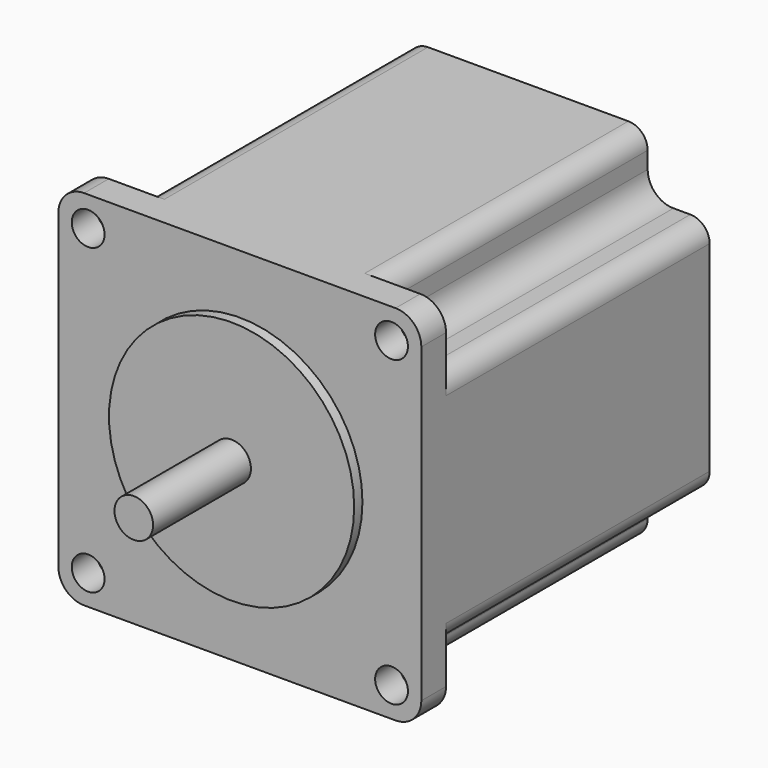
from build123d import *

# Parameters (mm, degrees)
F0_W     = 56.4
F0_H     = 56.4
F0_R     = 2.55
F0_R_2   = 19.05
F0_R_3   = 3
F1_DEPTH = 4.8
F2_DEPTH = 1.6
F3_DEPTH = 20.6
F4_R     = 4
F7_W     = 37.14
F7_H     = 9.63
F7_H_2   = 37.14
F7_W_2   = 9.63
F8_DEPTH = 56
F9_R     = 4
F10_R    = 3


# Not quite as in the source:
# - a feature of the source that left no trace in its solid (it failed there, or was rolled back) is left out


with BuildPart() as f1:
    # F0 (on Front) → F1 (new body)
    with BuildSketch(Plane.XZ):
        Rectangle(F0_W, F0_H)
        with Locations((-23.57, -23.57)):
            Circle(F0_R, mode=Mode.SUBTRACT)
        with Locations((23.57, -23.57)):
            Circle(F0_R, mode=Mode.SUBTRACT)
        with Locations((-23.57, 23.57)):
            Circle(F0_R, mode=Mode.SUBTRACT)
        Circle(F0_R_2, mode=Mode.SUBTRACT)
        with Locations((23.57, 23.57)):
            Circle(F0_R, mode=Mode.SUBTRACT)
        Circle(F0_R_2)
        Circle(F0_R_3, mode=Mode.SUBTRACT)
        Circle(F0_R_3)
    extrude(amount=-F1_DEPTH)

    # F4
    f4_edges = [f1.edges().sort_by_distance(p)[0] for p in [
        (-28.2, 2.4, 28.2),
        (28.2, 2.4, 28.2),
        (28.2, 2.4, -28.2),
        (-28.2, 2.4, -28.2),
    ]]
    fillet(f4_edges, radius=F4_R)

    # F7 (on Front) → F8 (join)
    with BuildSketch(Plane.XZ):
        with Locations((0, 23.385)):
            Rectangle(F7_W, F7_H)
        Rectangle(F7_W, F7_H_2)
        with Locations((-23.385, 0)):
            Rectangle(F7_W_2, F7_H_2)
        with Locations((23.385, 0)):
            Rectangle(F7_W_2, F7_H_2)
        with Locations((0, -23.385)):
            Rectangle(F7_W, F7_H)
    extrude(amount=-F8_DEPTH)

    # F9
    f9_edges = [f1.edges().sort_by_distance(p)[0] for p in [
        (18.57, 30.4, 18.57),
        (-18.57, 30.4, 18.57),
        (-18.57, 30.4, -18.57),
        (18.57, 30.4, -18.57),
    ]]
    fillet(f9_edges, radius=F9_R)

    # F10
    f10_edges = [f1.edges().sort_by_distance(p)[0] for p in [
        (18.57, 30.4, 28.2),
        (28.2, 30.4, 18.57),
        (28.2, 30.4, -18.57),
        (18.57, 30.4, -28.2),
        (-18.57, 30.4, -28.2),
        (-28.2, 30.4, -18.57),
        (-28.2, 30.4, 18.57),
        (-18.57, 30.4, 28.2),
    ]]
    fillet(f10_edges, radius=F10_R)


with BuildPart() as f2:
    # F0 (on Front) → F2 (new body)
    with BuildSketch(Plane.XZ):
        Circle(F0_R_2)
        Circle(F0_R_3, mode=Mode.SUBTRACT)
    extrude(amount=F2_DEPTH)


with BuildPart() as f3:
    # F0 (on Front) → F3 (new body)
    with BuildSketch(Plane.XZ):
        Circle(F0_R_3)
    extrude(amount=F3_DEPTH)


solid = Compound([f1.part, f2.part, f3.part])
